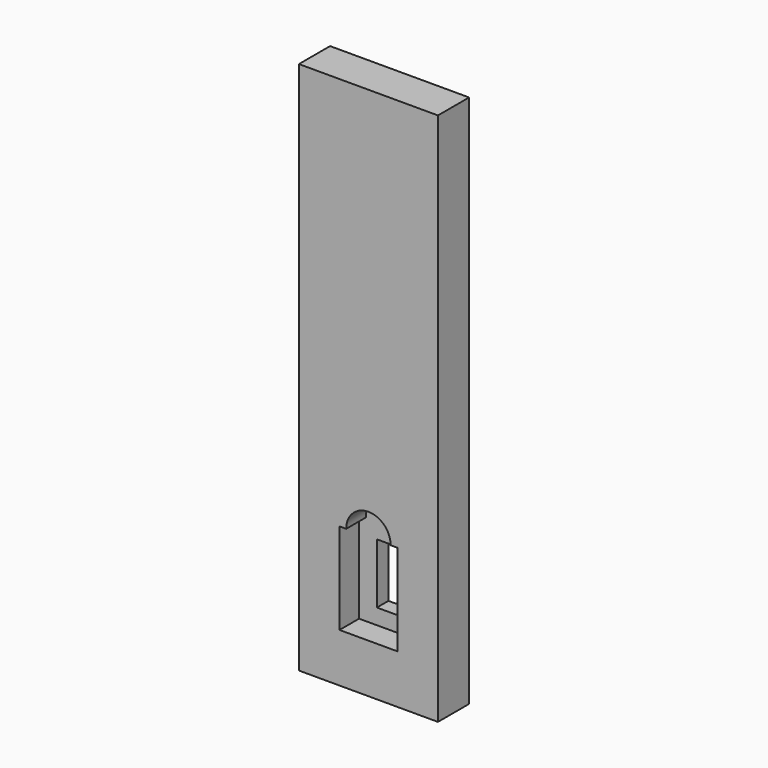
from build123d import *

# Parameters (mm, degrees)
F0_W     = 12.5
F0_H     = 48
F1_DEPTH = 3.5
F2_W     = 5.2
F2_H     = 8.2
F3_DEPTH = 2.2
F4_W     = 2
F4_H     = 5.4
F5_DEPTH = 3.5
F6_R     = 2
F7_DEPTH = 2.2


# Not quite as in the source:
# - a feature names something its author has since deleted; it is built from what else it names


with BuildPart() as f1:
    # F0 (on Front) → F1 (new body)
    with BuildSketch(Plane.XZ):
        Rectangle(F0_W, F0_H)
    extrude(amount=-F1_DEPTH)

    # F2 (on Front) → F3 (cut)
    with BuildSketch(Plane.XZ):
        with Locations((0, -15.5)):
            Rectangle(F2_W, F2_H)
    extrude(amount=-F3_DEPTH, mode=Mode.SUBTRACT)

    # F4 (on Front) → F5 (cut)
    with BuildSketch(Plane.XZ):
        with Locations((0, -15.5)):
            Rectangle(F4_W, F4_H)
    extrude(amount=-F5_DEPTH, mode=Mode.SUBTRACT)

    # F6 (on Front) → F7 (cut)
    with BuildSketch(Plane.XZ):
        with Locations((0, -11.4)):
            Circle(F6_R)
    extrude(amount=-F7_DEPTH, mode=Mode.SUBTRACT)


solid = f1.part
